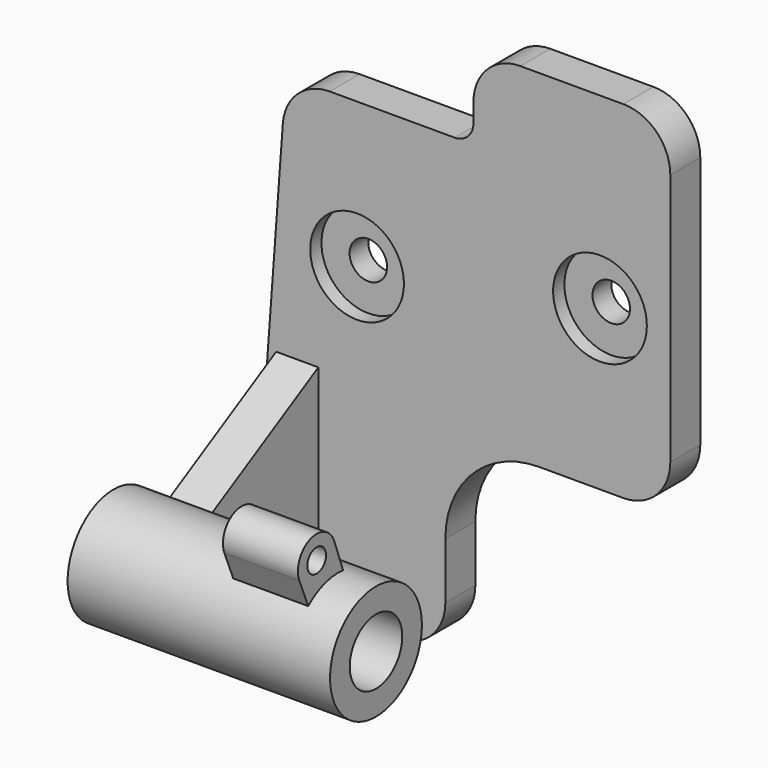
from build123d import *

# Parameters (mm, degrees)
F0_R           = 2
F1_DEPTH       = 4
F2_R           = 5
F3_DEPTH       = 1.5
F4_R           = 6.125
F4_R_2         = 3.5
F5_DEPTH       = 20
F6_R           = 1.25
F7_DEPTH       = 8
F8_DEPTH       = 4
F10_DEPTH      = 3.5
F10_DEPTH_BACK = 1
F11_DEPTH      = 4


with BuildPart() as f1:
    # F0 (on Front) → F1 (new body)
    with BuildSketch(Plane.XZ):
        with BuildLine():
            ThreePointArc((-3, -10), (-0.0710678119, -2.9289321881), (7, 0))
            Line((7, 0), (16, 0))
            ThreePointArc((16, 0), (19.5355339059, 1.4644660941), (21, 5))
            Line((21, 5), (21, 32))
            ThreePointArc((21, 32), (19.5355339059, 35.5355339059), (16, 37))
            Line((16, 37), (5, 37))
            ThreePointArc((5, 37), (1.4644660941, 35.5355339059), (0, 32))
            Line((0, 32), (0, 30))
            ThreePointArc((0, 30), (-0.5857864376, 28.5857864376), (-2, 28))
            Line((-2, 28), (-15.3529466806, 28))
            ThreePointArc((-15.3529466806, 28), (-18.7568523372, 26.6624344747), (-20.3395792507, 23.3653705126))
            Line((-20.3395792507, 23.3653705126), (-23.2757329417, -16.7077035899))
            ThreePointArc((-23.2757329417, -16.7077035899), (-22.2163744655, -19.7231245252), (-19.2864268857, -21))
            Line((-19.2864268857, -21), (-8, -21))
            ThreePointArc((-8, -21), (-4.4644660941, -19.5355339059), (-3, -16))
            Line((-3, -16), (-3, -10))
        make_face()
        with Locations((-12.4181403654, 12.5)):
            Circle(F0_R, mode=Mode.SUBTRACT)
        with Locations((13.5, 17)):
            Circle(F0_R, mode=Mode.SUBTRACT)
    extrude(amount=F1_DEPTH)

    # F2 (on face) → F3 (cut)
    with BuildSketch(Plane.XZ.offset(4)):
        with Locations((-12.4181403654, 12.5)):
            Circle(F2_R)
        with Locations((13.5, 17)):
            Circle(F2_R)
    extrude(amount=-F3_DEPTH, mode=Mode.SUBTRACT)


with BuildPart() as f5:
    # F4 (on Right) → F5 (new body)
    with BuildSketch(Plane.YZ):
        with Locations((-22, -11)):
            Circle(F4_R)
        with Locations((-22, -11)):
            Circle(F4_R_2, mode=Mode.SUBTRACT)
    extrude(amount=-F5_DEPTH)

    # F4 (on Right) → F8 (join)
    with BuildSketch(Plane.YZ):
        with Locations((-22, -11)):
            Circle(F4_R)
        with Locations((-22, -11)):
            Circle(F4_R_2, mode=Mode.SUBTRACT)
    extrude(amount=F8_DEPTH)

    # F11 (add): a face of the model
    f11_faces = [f5.faces().sort_by_distance(p)[0] for p in [
        (-20, -27.9517588386, -11),
    ]]
    extrude(f11_faces, amount=F11_DEPTH)


with BuildPart() as f7:
    # F6 (on face) → F7 (new body)
    with BuildSketch(Plane.YZ):
        with BuildLine():
            ThreePointArc((-27.2245328288, -3.5167956513), (-24.4274190035, -5.0149827659), (-22.4137369271, -2.56273994))
            ThreePointArc((-22.4137369271, -2.56273994), (-22.4522212571, -2.125772428), (-22.5664894122, -1.7022580377))
            ThreePointArc((-22.5664894122, -1.7022580377), (-25.8211887813, -0.2332483362), (-27.2245328288, -3.5167956513))
        make_face()
        with Locations((-24.9137369271, -2.56273994)):
            Circle(F6_R, mode=Mode.SUBTRACT)
        with BuildLine():
            ThreePointArc((-22.5664894122, -1.7022580377), (-22.4522212571, -2.125772428), (-22.4137369271, -2.56273994))
            ThreePointArc((-22.4137369271, -2.56273994), (-24.4274190035, -5.0149827659), (-27.2245328288, -3.5167956513))
            Line((-27.2245328288, -3.5167956513), (-26.0368237989, -6.3935177612))
            ThreePointArc((-26.0368237989, -6.3935177612), (-23.8690895414, -5.1671508432), (-21.3923093478, -4.9052205068))
            Line((-21.3923093478, -4.9052205068), (-22.5664894122, -1.7022580377))
        make_face()
    extrude(amount=-F7_DEPTH)


with BuildPart() as f10:
    # F9 (on face) → F10 (new body, two sides)
    with BuildSketch(Plane(origin=(-20, 0, 0), x_dir=(0, -1, 0), z_dir=(-1, 0, 0))) as f10_sk:
        with BuildLine():
            Line((4, -21), (23.1384048777, -17.0182771068))
            ThreePointArc((23.1384048777, -17.0182771068), (16.4200946717, -13.5259219163), (18.2291235039, -6.1733950388))
            Line((18.2291235039, -6.1733950388), (4.0624700915, 1.7376900148))
            Line((4.0624700915, 1.7376900148), (4, -21))
        make_face()
    extrude(amount=-F10_DEPTH)
    extrude(f10_sk.sketch, amount=F10_DEPTH_BACK)


with BuildPart() as f5_1:
    # F12: moved
    add(f5.part)


with BuildPart() as f7_1:
    # F12: moved
    add(f7.part)


with BuildPart() as f10_1:
    # F12: moved
    add(f10.part)


solid = Compound([f1.part, f5_1.part, f7_1.part, f10_1.part])
